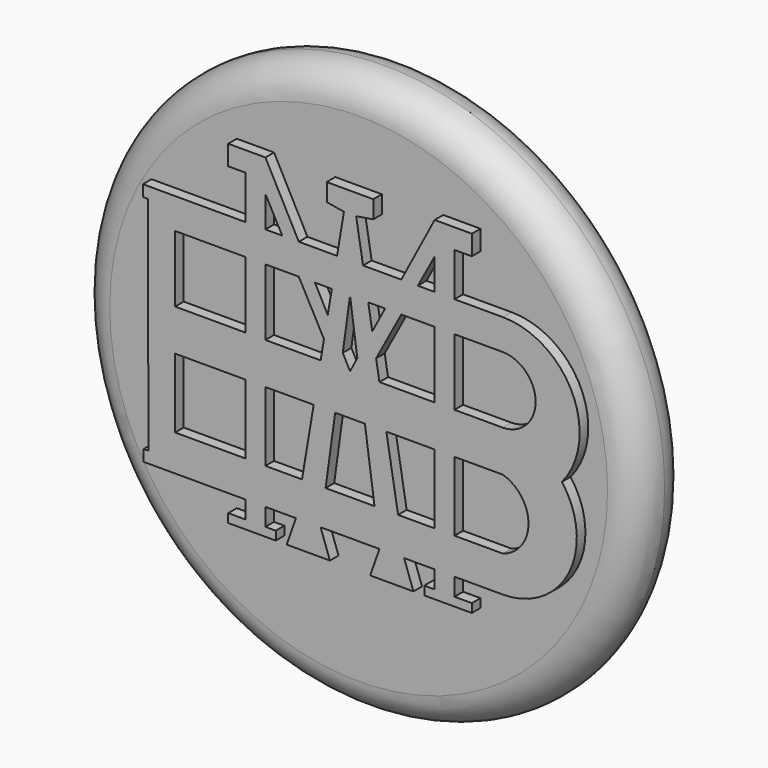
from build123d import *

# Parameters (mm, degrees)
F0_R     = 11.25
F0_R_2   = 6.1
F0_R_3   = 4.125
F1_DEPTH = 2.54
F2_DEPTH = 4.25
F3_DEPTH = 1
F5_W     = 2.82376213
F5_H     = 0.5161568988
F5_W_2   = 0.7975271437
F5_H_2   = 2.7843180578
F5_H_3   = 2.6690037921
F5_H_4   = 1.2320959941
F5_H_5   = 1.4468301088
F5_H_6   = 1.1431314051
F6_DEPTH = 0.4318


# Not quite as in the source:
# - a fillet or chamfer that OpenCascade refuses, or shapes differently, is made with other operations: its cross-section is extruded or revolved along the edge and cut away or added


with BuildPart() as f1:
    # F0 (on Front) → F1 (new body)
    with BuildSketch(Plane.XZ):
        Circle(F0_R)
        Circle(F0_R_2, mode=Mode.SUBTRACT)
        Circle(F0_R_2)
        Circle(F0_R_3, mode=Mode.SUBTRACT)
        Circle(F0_R_3)
    extrude(amount=F1_DEPTH)

    # F0 (on Front) → F2 (join)
    with BuildSketch(Plane.XZ):
        Circle(F0_R_3)
    extrude(amount=-F2_DEPTH)

    # F0 (on Front) → F3 (join)
    with BuildSketch(Plane.XZ):
        Circle(F0_R_2)
        Circle(F0_R_3, mode=Mode.SUBTRACT)
    extrude(amount=-F3_DEPTH)

    # F4: fillet of radius 1.27 on 3 edges, made by hand

    # F4_s1 → F4_t2 (revolve, cut)
    with BuildSketch(Plane.XY):
        with BuildLine():
            ThreePointArc((6.1, 0), (5.6559015079, 0.7188882647), (4.8590326354, 1))
            Line((4.8590326354, 1), (6.1, 1))
            Line((6.1, 1), (6.1, 0))
        make_face()
    revolve(axis=Axis((0, 1, 0), (0, -1, 0)), mode=Mode.SUBTRACT)

    # F4_s3 → F4_t4 (revolve, cut)
    with BuildSketch(Plane.XY):
        with BuildLine():
            ThreePointArc((11.25, -1.27), (10.8780256121, -0.3719743879), (9.98, 0))
            Line((9.98, 0), (11.25, 0))
            Line((11.25, 0), (11.25, -1.27))
        make_face()
    revolve(axis=Axis((0, 0, 0), (0, -1, 0)), mode=Mode.SUBTRACT)

    # F4_s5 → F4_t6 (revolve, cut)
    with BuildSketch(Plane.XY):
        with BuildLine():
            ThreePointArc((11.25, -1.27), (10.8780256121, -2.1680256121), (9.98, -2.54))
            Line((9.98, -2.54), (11.25, -2.54))
            Line((11.25, -2.54), (11.25, -1.27))
        make_face()
    revolve(axis=Axis((0, -2.54, 0), (0, -1, 0)), mode=Mode.SUBTRACT)

    # F5 (on face) → F6 (join)
    with BuildSketch(Plane.XZ.offset(2.54)):
        with Locations((-5.6011655834, -0.2580784494)):
            Rectangle(F5_W, F5_H)
        Polygon((-2.7183012693, 5.0442311913), (-2.0541941821, 5.0442311913), (-3.3917573746, 7.5843841769), (-4.882786423, 7.5843841769), (-4.882786423, 6.7868568003), (-4.1892845184, 6.7868568003), (-4.1892845184, 5.0442311913), (-3.3917573746, 5.0442311913), (-3.3917573746, 6.2939338386), align=None)
        Polygon((-0.3677175585, 1.1431314051), (0, 1.1431314051), (-0.2914590528, 1.6966384), align=None)
        Polygon((3.3917573746, 5.0442311913), (4.1892845184, 5.0442311913), (4.1892845184, 6.7868568003), (4.882786423, 6.7868568003), (4.882786423, 7.5843841769), (3.3917573746, 7.5843841769), (2.0541941821, 5.0442311913), (2.7183012693, 5.0442311913), (3.3917573746, 6.2939338386), align=None)
        Polygon((-0.521645051, 5.0442311913), (0.521645051, 5.0442311913), (0.2444440033, 6.6919331439), (0.9331664045, 6.8078003193), (0.9331664045, 7.516650483), (0, 7.516650483), (-0.9331664045, 7.516650483), (-0.9331664045, 6.8078003193), (-0.2444440033, 6.6919331439), align=None)
        Polygon((0.6160256007, 1.1431314051), (1.1779463597, 1.1431314051), (1.0442581093, 1.9377834924), align=None)
        Polygon((0, 1.1431314051), (0.3677175585, 1.1431314051), (0.2914590528, 1.6966384), align=None)
        with BuildLine():
            ThreePointArc((6.1259130016, 3.8121351972), (7.4410236088, 2.4776333012), (6.1259130016, 1.1431314051))
            Line((6.1259130016, 1.1431314051), (4.1892845184, 1.1431314051))
            Line((4.1892845184, 1.1431314051), (4.1892845184, 0))
            Line((4.1892845184, 0), (8.4969736636, 0))
            ThreePointArc((8.4969736636, 0), (8.9127659298, 3.2748235651), (6.1259130016, 5.0442311913))
            Line((6.1259130016, 5.0442311913), (5.1765339449, 5.0442311913))
            Line((5.1765339449, 5.0442311913), (4.1892845184, 5.0442311913))
            Line((4.1892845184, 5.0442311913), (4.1892845184, 3.8121351972))
            Line((4.1892845184, 3.8121351972), (6.1259130016, 3.8121351972))
        make_face()
        Polygon((-3.3917573746, -5.4534515366), (-3.3917573746, -4.7473050654), (-4.1892845184, -4.7473050654), (-4.1892845184, -5.4534515366), (-4.882786423, -5.4534515366), (-4.882786423, -5.8025359176), (-2.9781798366, -5.8025359176), (-2.9781798366, -5.4534515366), align=None)
        Polygon((-0.8081396227, -5.8025359176), (-1.1792626465, -4.7473050654), (-2.1689236164, -4.7473050654), (-2.5400463492, -5.8025359176), align=None)
        Polygon((2.5400463492, -5.8025359176), (2.1689236164, -4.7473050654), (1.1792626465, -4.7473050654), (0.8081396227, -5.8025359176), align=None)
        Polygon((4.1892845184, -5.4534515366), (4.1892845184, -4.7473050654), (3.3917573746, -4.7473050654), (3.3917573746, -5.4534515366), (2.9781798366, -5.4534515366), (2.9781798366, -5.8025359176), (4.882786423, -5.8025359176), (4.882786423, -5.4534515366), align=None)
        with Locations((-3.7905209465, -1.9083159277)):
            Rectangle(F5_W_2, F5_H_2)
        with Locations((-3.7905209465, -0.2580784494)):
            Rectangle(F5_W_2, F5_H)
        with Locations((-3.7905209465, 2.4776333012)):
            Rectangle(F5_W_2, F5_H_3)
        with Locations((-3.7905209465, 4.4281831942)):
            Rectangle(F5_W_2, F5_H_4)
        Polygon((-0.3677175585, 1.1431314051), (-0.2914590528, 1.6966384), (-0.8927262809, 2.8384990261), (-1.0442581093, 1.9377834924), (-0.6160256007, 1.1431314051), align=None)
        Polygon((-1.0442581093, 1.9377834924), (-0.8927262809, 2.8384990261), (-1.4054118998, 3.8121351972), (-2.0543332675, 3.8121351972), align=None)
        Polygon((-0.2914590528, 1.6966384), (0, 3.8121351972), (-0.728926653, 3.8121351972), (-0.8927262809, 2.8384990261), align=None)
        Polygon((0.2914590528, 1.6966384), (0.8927262809, 2.8384990261), (0.728926653, 3.8121351972), (0, 3.8121351972), align=None)
        Polygon((0.6160256007, 1.1431314051), (1.0442581093, 1.9377834924), (0.8927262809, 2.8384990261), (0.2914590528, 1.6966384), (0.3677175585, 1.1431314051), align=None)
        Polygon((0, 0), (0.4182745639, 0.7761735704), (0.3677175585, 1.1431314051), (0, 1.1431314051), (-0.3677175585, 1.1431314051), (-0.4182745639, 0.7761735704), align=None)
        with Locations((3.7905209465, -1.9083159277)):
            Rectangle(F5_W_2, F5_H_2)
        with Locations((3.7905209465, -0.2580784494)):
            Rectangle(F5_W_2, F5_H)
        with Locations((3.7905209465, 2.4776333012)):
            Rectangle(F5_W_2, F5_H_3)
        with Locations((3.7905209465, 4.4281831942)):
            Rectangle(F5_W_2, F5_H_4)
        Polygon((1.0442581093, 1.9377834924), (2.0543332675, 3.8121351972), (1.4054118998, 3.8121351972), (0.8927262809, 2.8384990261), align=None)
        Polygon((-0.6160256007, 1.1431314051), (-0.4182745639, 0.7761735704), (-0.3677175585, 1.1431314051), align=None)
        Polygon((0.4182745639, 0.7761735704), (0.6160256007, 1.1431314051), (0.3677175585, 1.1431314051), align=None)
        Polygon((-1.4054118998, 3.8121351972), (-2.0541941821, 5.0442311913), (-2.7183012693, 5.0442311913), (-2.0543332675, 3.8121351972), align=None)
        Polygon((1.4054118998, 3.8121351972), (2.0543332675, 3.8121351972), (2.7183012693, 5.0442311913), (2.0541941821, 5.0442311913), align=None)
        Polygon((-8.0940451721, 0), (-7.0130466484, 0), (-7.0130466484, 1.1431314051), (-7.0130466484, 3.8121351972), (-4.1892845184, 3.8121351972), (-4.1892845184, 5.0442311913), (-7.7138240449, 5.0442311913), (-8.3028590307, 5.0442311913), (-8.3028590307, 4.5893052593), (-8.1096682698, 4.5893052593), align=None)
        Polygon((2.0543332675, 3.8121351972), (3.3917573746, 3.8121351972), (3.3917573746, 5.0442311913), (2.7183012693, 5.0442311913), align=None)
        with Locations((-3.7905209465, -4.023890011)):
            Rectangle(F5_W_2, F5_H_5)
        Polygon((-2.0543332675, 3.8121351972), (-2.7183012693, 5.0442311913), (-3.3917573746, 5.0442311913), (-3.3917573746, 3.8121351972), align=None)
        Polygon((-0.728926653, 3.8121351972), (-0.521645051, 5.0442311913), (-2.0541941821, 5.0442311913), (-1.4054118998, 3.8121351972), align=None)
        Polygon((0, 3.8121351972), (0.728926653, 3.8121351972), (0.521645051, 5.0442311913), (-0.521645051, 5.0442311913), (-0.728926653, 3.8121351972), align=None)
        Polygon((0.728926653, 3.8121351972), (1.4054118998, 3.8121351972), (2.0541941821, 5.0442311913), (0.521645051, 5.0442311913), align=None)
        Polygon((-1.1779463597, 1.1431314051), (-0.6160256007, 1.1431314051), (-1.0442581093, 1.9377834924), align=None)
        Polygon((1.4570966365, -0.5161568988), (1.370261009, 0), (0.5252105866, 0), (0.5963232449, -0.5161568988), align=None)
        Polygon((3.3917573746, -0.5161568988), (3.3917573746, 0), (1.370261009, 0), (1.4570966365, -0.5161568988), align=None)
        Polygon((-3.3917573746, -0.5161568988), (-1.4570966365, -0.5161568988), (-1.370261009, 0), (-3.3917573746, 0), align=None)
        Polygon((-1.4570966365, -0.5161568988), (-0.5963232449, -0.5161568988), (-0.5252105866, 0), (-1.370261009, 0), align=None)
        Polygon((-0.9799280345, -3.3004749566), (-0.5963232449, -0.5161568988), (-1.4570966365, -0.5161568988), (-1.9255162324, -3.3004749566), align=None)
        Polygon((1.9255162324, -3.3004749566), (1.4570966365, -0.5161568988), (0.5963232449, -0.5161568988), (0.9799280345, -3.3004749566), align=None)
        Polygon((2.1689236164, -4.7473050654), (1.9255162324, -3.3004749566), (0.9799280345, -3.3004749566), (1.1792626465, -4.7473050654), align=None)
        Polygon((3.3917573746, -4.7473050654), (3.3917573746, -3.3004749566), (1.9255162324, -3.3004749566), (2.1689236164, -4.7473050654), align=None)
        with Locations((3.7905209465, -4.023890011)):
            Rectangle(F5_W_2, F5_H_5)
        Polygon((-1.1792626465, -4.7473050654), (-0.9799280345, -3.3004749566), (-1.9255162324, -3.3004749566), (-2.1689236164, -4.7473050654), align=None)
        Polygon((-2.1689236164, -4.7473050654), (-1.9255162324, -3.3004749566), (-3.3917573746, -3.3004749566), (-3.3917573746, -4.7473050654), align=None)
        Polygon((1.1792626465, -4.7473050654), (0.9799280345, -3.3004749566), (-0.9799280345, -3.3004749566), (-1.1792626465, -4.7473050654), align=None)
        Polygon((0.5963232449, -0.5161568988), (0.5252105866, 0), (0, 0), (-0.5252105866, 0), (-0.5963232449, -0.5161568988), align=None)
        with Locations((-5.6011655834, 0.5715657026)):
            Rectangle(F5_W, F5_H_6)
        with Locations((-3.7905209465, 0.5715657026)):
            Rectangle(F5_W_2, F5_H_6)
        Polygon((-3.3917573746, 0), (-1.370261009, 0), (-1.1779463597, 1.1431314051), (-3.3917573746, 1.1431314051), align=None)
        Polygon((-0.5252105866, 0), (-0.4182745639, 0.7761735704), (-0.6160256007, 1.1431314051), (-1.1779463597, 1.1431314051), (-1.370261009, 0), align=None)
        Polygon((-0.5252105866, 0), (0, 0), (-0.4182745639, 0.7761735704), align=None)
        Polygon((0, 0), (0.5252105866, 0), (0.4182745639, 0.7761735704), align=None)
        Polygon((1.370261009, 0), (1.1779463597, 1.1431314051), (0.6160256007, 1.1431314051), (0.4182745639, 0.7761735704), (0.5252105866, 0), align=None)
        Polygon((3.3917573746, 0), (3.3917573746, 1.1431314051), (1.1779463597, 1.1431314051), (1.370261009, 0), align=None)
        with Locations((3.7905209465, 0.5715657026)):
            Rectangle(F5_W_2, F5_H_6)
        with BuildLine():
            Line((8.4969736636, 0), (4.1892845184, 0))
            Line((4.1892845184, 0), (4.1892845184, -0.5161568988))
            Line((4.1892845184, -0.5161568988), (6.1259130016, -0.5161568988))
            ThreePointArc((6.1259130016, -0.5161568988), (7.1544234466, -1.9083159277), (6.1259130016, -3.3004749566))
            Line((6.1259130016, -3.3004749566), (4.1892845184, -3.3004749566))
            Line((4.1892845184, -3.3004749566), (4.1892845184, -4.7473050654))
            Line((4.1892845184, -4.7473050654), (6.1259130016, -4.7473050654))
            ThreePointArc((6.1259130016, -4.7473050654), (8.7791579039, -3.106708495), (8.4969736636, 0))
        make_face()
        Polygon((-4.1892845184, -4.7473050654), (-4.1892845184, -3.3004749566), (-7.0130466484, -3.3004749566), (-7.0130466484, -0.5161568988), (-7.0130466484, 0), (-8.0940451721, 0), (-8.0794328824, -4.2923791334), (-8.2726236433, -4.2923791334), (-8.2726236433, -4.7473050654), (-7.7138240449, -4.7473050654), (-7.6835886575, -4.7473050654), align=None)
    extrude(amount=F6_DEPTH)


solid = f1.part
